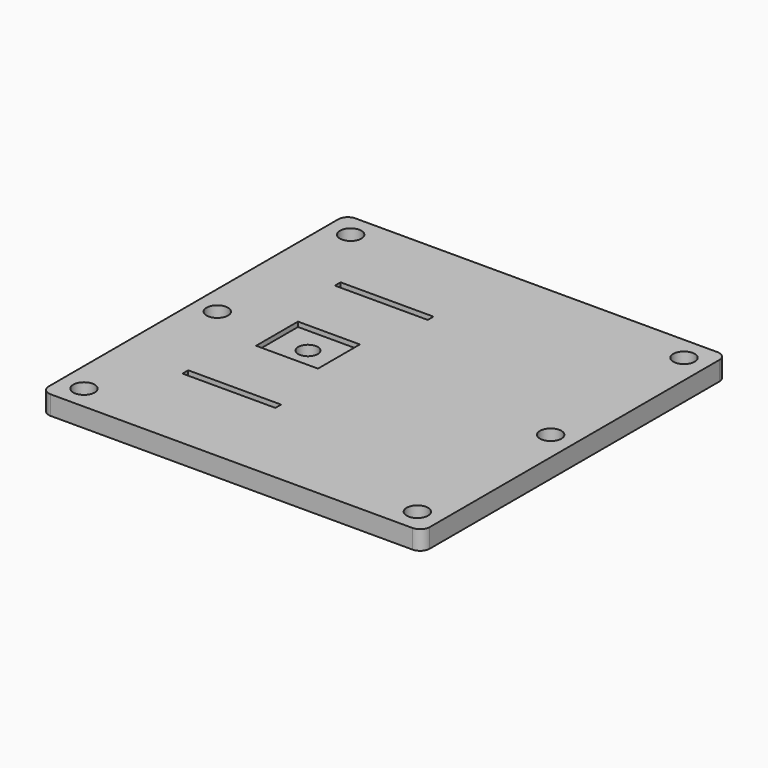
from build123d import *

# Parameters (mm, degrees)
F0_R     = 2.25
F1_DEPTH = 4
F2_R     = 2.05
F3_DEPTH = 5
F4_W     = 13
F4_H     = 11
F5_DEPTH = 1
F6_W     = 19.5
F6_H     = 1.5
F7_DEPTH = 25


# Not quite as in the source:
# - a feature names something its author has since deleted; it is built from what else it names


with BuildPart() as f1:
    # F0 (on Top) → F1 (new body)
    with BuildSketch(Plane.XY):
        with BuildLine():
            ThreePointArc((40, 38), (39.4142135624, 39.4142135624), (38, 40))
            Line((38, 40), (-38, 40))
            ThreePointArc((-38, 40), (-39.4142135624, 39.4142135624), (-40, 38))
            Line((-40, 38), (-40, -38))
            ThreePointArc((-40, -38), (-39.4142135624, -39.4142135624), (-38, -40))
            Line((-38, -40), (38, -40))
            ThreePointArc((38, -40), (39.4142135624, -39.4142135624), (40, -38))
            Line((40, -38), (40, 38))
        make_face()
        with Locations((-35, -35)):
            Circle(F0_R, mode=Mode.SUBTRACT)
        with Locations((35, -35)):
            Circle(F0_R, mode=Mode.SUBTRACT)
        with Locations((-35, 0)):
            Circle(F0_R, mode=Mode.SUBTRACT)
        with Locations((-35, 35)):
            Circle(F0_R, mode=Mode.SUBTRACT)
        with Locations((35, 0)):
            Circle(F0_R, mode=Mode.SUBTRACT)
        with Locations((35, 35)):
            Circle(F0_R, mode=Mode.SUBTRACT)
    extrude(amount=F1_DEPTH)

    # F2 (on face) → F3 (cut)
    with BuildSketch(Plane.XY.offset(4)):
        with Locations((-15.9661, 0)):
            Circle(F2_R)
    extrude(amount=-F3_DEPTH, mode=Mode.SUBTRACT)

    # F4 (on face) → F5 (cut)
    with BuildSketch(Plane.XY.offset(4)):
        with Locations((-15.9661, 0)):
            Rectangle(F4_W, F4_H)
    extrude(amount=-F5_DEPTH, mode=Mode.SUBTRACT)

    # F6 (on face) → F7 (cut)
    with BuildSketch(Plane.XY.offset(4)):
        with Locations((-15.9661, 20)):
            Rectangle(F6_W, F6_H)
        with Locations((-15.9661, -20)):
            Rectangle(F6_W, F6_H)
    extrude(amount=-F7_DEPTH, mode=Mode.SUBTRACT)


solid = f1.part
